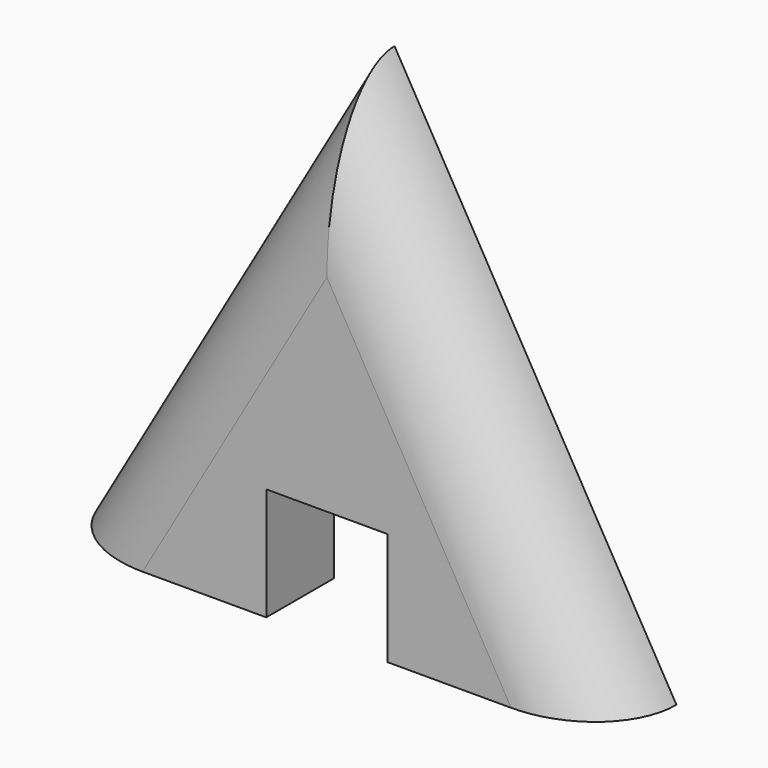
from build123d import *

# Parameters (mm, degrees)
F1_DEPTH = 3
F2_R     = 2.99999


# Not quite as in the source:
# - a fillet or chamfer is up to 0.001 mm smaller than in the source, because OpenCascade refuses the exact size


with BuildPart() as f1:
    # F0 (on Front) → F1 (new body)
    with BuildSketch(Plane.XZ):
        Polygon((0, 17.3205080757), (-10, 0), (-2.15, 0), (-2.15, 4), (2.15, 4), (2.15, 0), (10, 0), align=None)
    extrude(amount=F1_DEPTH)

    # F2 (radius 3 in the source; OpenCascade refuses exactly that, so slightly less here)
    f2_edges = [f1.edges().sort_by_distance(p)[0] for p in [
        (-5, -3, 8.660254),
        (5, -3, 8.660254),
    ]]
    fillet(f2_edges, radius=F2_R)


solid = f1.part
